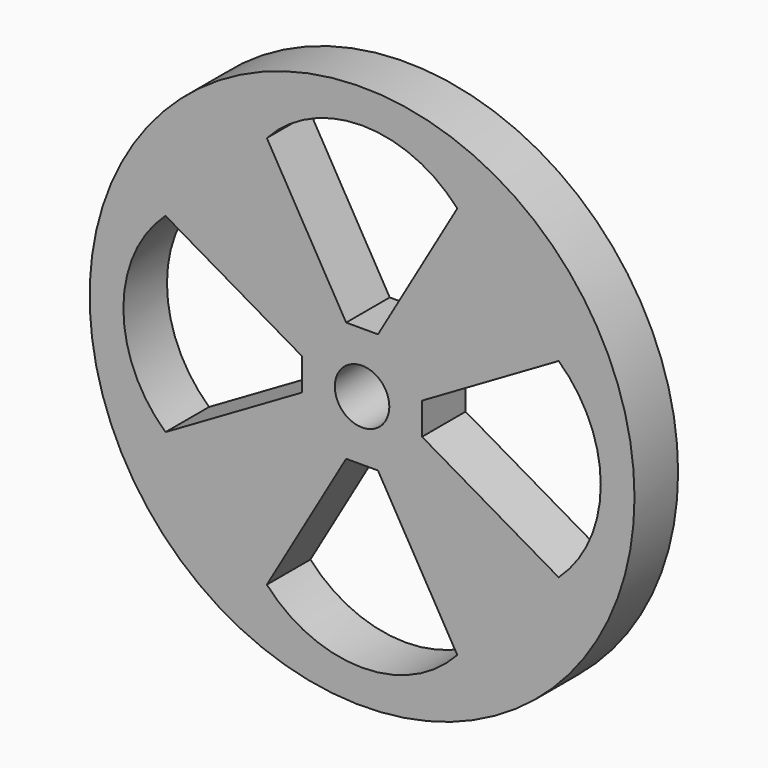
from build123d import *

# Parameters (mm, degrees)
F0_R            = 63.5
F1_DEPTH        = 12.7
F2_R            = 6.35
F3_DEPTH        = 12.701
F5_DEPTH        = 12.701
F5_COPIES_COUNT = 4


# Not quite as in the source:
# - a pattern or mirror of a feature is missing from the dataset's text; its kind, count and spacing are read off the source's solid


with BuildPart() as f1:
    # F0 (on Front) → F1 (new body)
    with BuildSketch(Plane.XZ):
        Circle(F0_R)
    extrude(amount=F1_DEPTH)

    # F2 (on face) → F3 (cut, through all)
    with BuildSketch(Plane.XZ.offset(12.7)):
        Circle(F2_R)
    extrude(amount=-F3_DEPTH, mode=Mode.SUBTRACT)

    # F4 (on face) → F5 (cut, through all)
    with BuildSketch(Plane.XZ.offset(12.7)):
        with BuildLine():
            Line((-22.1979282796, 45.8192452788), (-3.7104284856, 13.9721687883))
            Line((-3.7104284856, 13.9721687883), (3.7104284856, 13.9721687883))
            Line((3.7104284856, 13.9721687883), (22.1979282796, 45.8192452788))
            ThreePointArc((22.1979282796, 45.8192452788), (0, 55.6319138023), (-22.1979282796, 45.8192452788))
        make_face()
    f5 = extrude(amount=-F5_DEPTH, mode=Mode.SUBTRACT)

    # F5_copies: F5 ×4 about axis
    f5_copies_axis = Axis((0, 0, 0), (0, 1, 0))
    for i in range(1, F5_COPIES_COUNT):
        add(f5.rotate(f5_copies_axis, i * 360 / F5_COPIES_COUNT), mode=Mode.SUBTRACT)


solid = f1.part
